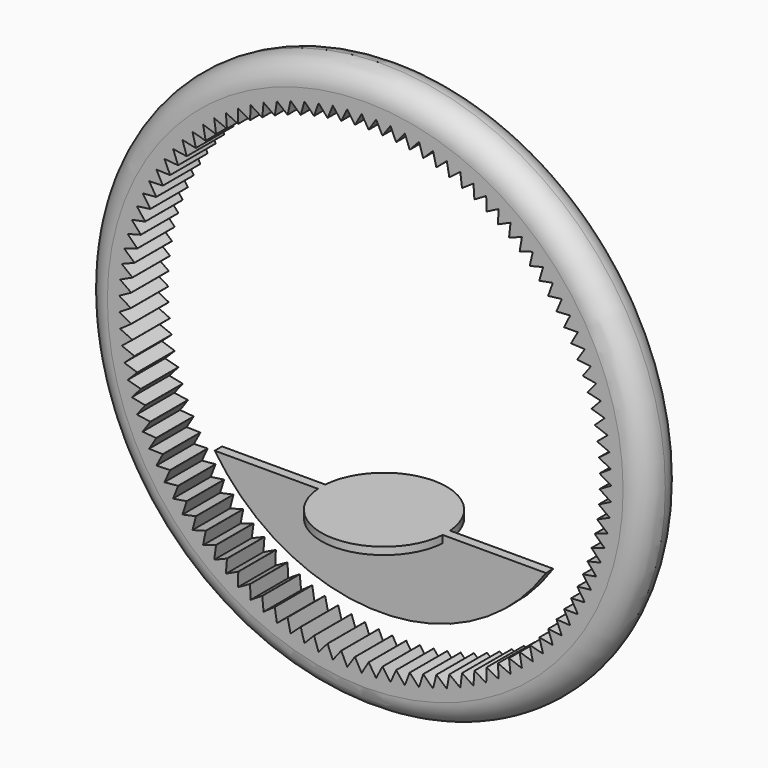
from build123d import *

# Parameters (mm, degrees)
F0_R          = 152.4
F1_DEPTH      = 12.7
F1_DEPTH_BACK = 12.7
F2_R          = 12.69999
F4_DEPTH      = 2.5
F6_DEPTH      = 4


# Not quite as in the source:
# - a fillet or chamfer is up to 0.001 mm smaller than in the source, because OpenCascade refuses the exact size


with BuildPart() as f1:
    # F0 (on Front) → F1 (new body, two sides)
    with BuildSketch(Plane.XZ) as f1_sk:
        Circle(F0_R)
        with BuildLine():
            ThreePointArc((126.9443490301, 3.7592884063), (126.9452637908, 3.7282705209), (126.9461709726, 3.6972524128))
            Line((126.9461709726, 3.6972524128), (133.35, 0))
            Line((133.35, 0), (126.9461709726, -3.6972524128))
            ThreePointArc((126.9461709726, -3.6972524128), (126.9452637908, -3.7282705209), (126.9443490301, -3.7592884063))
            Line((126.9443490301, -3.7592884063), (133.1201574625, -7.825993685))
            Line((133.1201574625, -7.825993685), (126.5103831653, -11.141048037))
            ThreePointArc((126.5103831653, -11.141048037), (126.5076571684, -11.1719594418), (126.5049236186, -11.2028701796))
            Line((126.5049236186, -11.2028701796), (132.4314221649, -15.6250095484))
            Line((132.4314221649, -15.6250095484), (125.6384878592, -18.5464381606))
            ThreePointArc((125.6384878592, -18.5464381606), (125.6339524441, -18.5771363041), (125.6294095284, -18.6078333386))
            Line((125.6294095284, -18.6078333386), (131.2861683203, -23.3701627671))
            Line((131.2861683203, -23.3701627671), (124.333490658, -25.8878948698))
            ThreePointArc((124.333490658, -25.8878948698), (124.3271614593, -25.9182739292), (124.3208248379, -25.9486514412))
            Line((124.3208248379, -25.9486514412), (129.6883438562, -31.0347541933))
            Line((129.6883438562, -31.0347541933), (122.5998901574, -33.1401106423))
            ThreePointArc((122.5998901574, -33.1401106423), (122.5917889932, -33.1700658947), (122.5836805098, -33.2000191667))
            Line((122.5836805098, -33.2000191667), (127.6434568043, -38.5923623926))
            Line((127.6434568043, -38.5923623926), (120.4436624375, -40.2780855882))
            ThreePointArc((120.4436624375, -40.2780855882), (120.433817234, -40.3075137715), (120.4239648403, -40.3369395484))
            Line((120.4239648403, -40.3369395484), (125.158556314, -46.0169347239))
            Line((125.158556314, -46.0169347239), (117.8722404618, -47.2772136289))
            ThreePointArc((117.8722404618, -47.2772136289), (117.8606851576, -47.3060132982), (117.8491228169, -47.3348101432))
            Line((117.8491228169, -47.3348101432), (122.2422083521, -53.2828771483))
            Line((122.2422083521, -53.2828771483), (114.8944884547, -54.1133673203))
            ThreePointArc((114.8944884547, -54.1133673203), (114.8812628833, -54.1414391971), (114.8680304533, -54.1695078415))
            Line((114.8680304533, -54.1695078415), (118.9044661741, -60.3651424569))
            Line((118.9044661741, -60.3651424569), (111.5206713441, -60.7629810242))
            ThreePointArc((111.5206713441, -60.7629810242), (111.5058210969, -60.790228339), (111.4909641924, -60.8174720244))
            Line((111.4909641924, -60.8174720244), (115.1568356688, -67.2393166142))
            Line((115.1568356688, -67.2393166142), (107.7624193767, -67.2031321449))
            ThreePointArc((107.7624193767, -67.2031321449), (107.7459956454, -67.2294609705), (107.7295654814, -67.2557857823))
            Line((107.7295654814, -67.2557857823), (111.0122356949, -73.8817029178))
            Line((111.0122356949, -73.8817029178), (103.6326880254, -73.4116201471))
            ThreePointArc((103.6326880254, -73.4116201471), (103.6147474261, -73.4369397226), (103.5968006407, -73.4622549137))
            Line((103.5968006407, -73.4622549137), (106.484953547, -80.2694036859))
            Line((106.484953547, -80.2694036859), (99.1457133298, -79.3670430866))
            ThreePointArc((99.1457133298, -79.3670430866), (99.1263177075, -79.3912661302), (99.106916167, -79.4154844339))
            Line((99.106916167, -79.4154844339), (101.5905957048, -86.3803991908))
            Line((101.5905957048, -86.3803991908), (94.3169628212, -85.0488713869))
            ThreePointArc((94.3169628212, -85.0488713869), (94.2961790365, -85.0719143966), (94.2753896221, -85.0949523274))
            Line((94.2753896221, -85.0949523274), (96.3460340334, -92.1936235649))
            Line((96.3460340334, -92.1936235649), (89.1630822029, -90.4375186086))
            ThreePointArc((89.1630822029, -90.4375186086), (89.1409819019, -90.4593021505), (89.1188762789, -90.4810802918))
            Line((89.1188762789, -90.4810802918), (90.7693476236, -97.6890374197))
            Line((90.7693476236, -97.6890374197), (83.7018379691, -95.5144089684))
            ThreePointArc((83.7018379691, -95.5144089684), (83.6784973361, -95.5348579502), (83.6551517073, -95.5553012283))
            Line((83.6551517073, -95.5553012283), (84.8797604686, -102.8476969251))
            Line((84.8797604686, -102.8476969251), (77.95205616, -100.2620413737))
            ThreePointArc((77.95205616, -100.2620413737), (77.927555655, -100.2810853034), (77.9030504975, -100.3001232461))
            Line((77.9030504975, -100.3001232461), (78.6975751954, -107.6518191131))
            Line((78.6975751954, -107.6518191131), (71.9335574647, -104.6640497519))
            ThreePointArc((71.9335574647, -104.6640497519), (71.907981546, -104.6816229812), (71.8824013342, -104.6991899607))
            Line((71.8824013342, -104.6991899607), (72.2441030774, -112.0848431793))
            Line((72.2441030774, -112.0848431793), (65.6670888949, -108.7052594683))
            ThreePointArc((65.6670888949, -108.7052594683), (65.640525728, -108.7213014186), (65.6139586422, -108.7373368779))
            Line((65.6139586422, -108.7373368779), (65.5415905699, -116.1314875715))
            Line((65.5415905699, -116.1314875715), (59.174252266, -112.3717396357))
            ThreePointArc((59.174252266, -112.3717396357), (59.1467934197, -112.3861950071), (59.1193310421, -112.4006436687))
            Line((59.1193310421, -112.4006436687), (58.6131426221, -119.777802668))
            Line((58.6131426221, -119.777802668), (52.477429731, -115.6508511375))
            ThreePointArc((52.477429731, -115.6508511375), (52.4491698615, -115.6636700993), (52.4209068606, -115.6764821557))
            Line((52.4209068606, -115.6764821557), (51.4826430292, -123.0112188653))
            Line((51.4826430292, -123.0112188653), (45.5997066243, -118.531290197))
            ThreePointArc((45.5997066243, -118.531290197), (45.5707431493, -118.5424285597), (45.5417769536, -118.5535598449))
            Line((45.5417769536, -118.5535598449), (44.1746721006, -125.820589908))
            Line((44.1746721006, -125.820589908), (38.5647918824, -121.0031273442))
            ThreePointArc((38.5647918824, -121.0031273442), (38.535224645, -121.0125467113), (38.5056551069, -121.0219588537))
            Line((38.5056551069, -121.0219588537), (36.714421926, -128.1962313122))
            Line((36.714421926, -128.1962313122), (31.3969363138, -123.0578416441))
            ThreePointArc((31.3969363138, -123.0578416441), (31.3668672383, -123.0655095453), (31.3367962902, -123.0731700992))
            Line((31.3367962902, -123.0731700992), (29.1276095332, -130.1299537496))
            Line((29.1276095332, -130.1299537496), (24.1208490014, -124.6883500711))
            ThreePointArc((24.1208490014, -124.6883500711), (24.0903817423, -124.6942400735), (24.0599130449, -124.7001226313))
            Line((24.0599130449, -124.7001226313), (21.4403882362, -131.6150912786))
            Line((21.4403882362, -131.6150912786), (16.7616121256, -125.8890319247))
            ThreePointArc((16.7616121256, -125.8890319247), (16.7308517098, -125.8931237243), (16.7000902951, -125.8972080077))
            Line((16.7000902951, -125.8972080077), (13.6792574793, -132.6465243224))
            Line((13.6792574793, -132.6465243224), (9.3445945005, -126.655748206))
            ThreePointArc((9.3445945005, -126.655748206), (9.3136469654, -126.6580276974), (9.2826988744, -126.660299627))
            Line((9.2826988744, -126.660299627), (5.8709714881, -133.2206973176))
            Line((5.8709714881, -133.2206973176), (1.8953641223, -126.985855885))
            ThreePointArc((1.8953641223, -126.985855885), (1.8643361506, -126.9863152104), (1.8333080676, -126.9867669544))
            Line((1.8333080676, -126.9867669544), (-1.9575529581, -133.3356309709))
            Line((-1.9575529581, -133.3356309709), (-5.5603999687, -126.8782170122))
            ThreePointArc((-5.5603999687, -126.8782170122), (-5.5914014172, -126.8768545882), (-5.6224025318, -126.8754845893))
            Line((-5.6224025318, -126.8754845893), (-9.7793293137, -132.9909290823))
            Line((-9.7793293137, -132.9909290823), (-12.9969962092, -126.333202641))
            ThreePointArc((-12.9969962092, -126.333202641), (-13.027864266, -126.3300231642), (-13.058731545, -126.3268361451))
            Line((-13.058731545, -126.3268361451), (-17.5673942953, -132.1877799105))
            Line((-17.5673942953, -132.1877799105), (-20.3887891111, -125.352691549))
            ThreePointArc((-20.3887891111, -125.352691549), (-20.4194173678, -125.3477059796), (-20.4500444053, -125.3427129267))
            Line((-20.4500444053, -125.3427129267), (-25.2949008294, -130.9289520772))
            Line((-25.2949008294, -130.9289520772), (-27.7102976333, -123.940063761))
            ThreePointArc((-27.7102976333, -123.940063761), (-27.7405805078, -123.9332892854), (-27.7708617261, -123.9265074106))
            Line((-27.7708617261, -123.9265074106), (-32.9352106003, -129.2187850226))
            Line((-32.9352106003, -129.2187850226), (-34.936283019, -122.1001888975))
            ThreePointArc((-34.936283019, -122.1001888975), (-34.96611612, -122.0916488687), (-34.9959471334, -122.0831015507))
            Line((-34.9959471334, -122.0831015507), (-40.4619858773, -127.0631740469))
            Line((-40.4619858773, -127.0631740469), (-42.0418357997, -119.8394093885))
            ThreePointArc((-42.0418357997, -119.8394093885), (-42.0711162863, -119.8291332457), (-42.1003942611, -119.8188499488))
            Line((-42.1003942611, -119.8188499488), (-47.8492803068, -124.4695499876))
            Line((-47.8492803068, -124.4695499876), (-49.0024616629, -117.1655186092))
            ThreePointArc((-49.0024616629, -117.1655186092), (-49.0310885993, -117.1535417765), (-49.0597126083, -117.1415579493))
            Line((-49.0597126083, -117.1415579493), (-55.0716283545, -121.4468536043))
            Line((-55.0716283545, -121.4468536043), (-55.7941658894, -114.0877340151))
            ThreePointArc((-55.7941658894, -114.0877340151), (-55.8220405925, -114.074097779), (-55.8499119628, -114.0604547323))
            Line((-55.8499119628, -114.0604547323), (-62.1041330907, -118.0055047574))
            Line((-62.1041330907, -118.0055047574), (-62.3935360677, -110.6166653673))
            ThreePointArc((-62.3935360677, -110.6166653673), (-62.4205624476, -110.6014167347), (-62.4475851008, -110.586161499))
            Line((-62.4475851008, -110.586161499), (-68.9225520144, -114.1573664895))
            Line((-68.9225520144, -114.1573664895), (-68.7778228015, -106.7642781584))
            ThreePointArc((-68.7778228015, -106.7642781584), (-68.8039076928, -106.7474696946), (-68.8299884762, -106.7306548577))
            Line((-68.8299884762, -106.7306548577), (-75.5033806233, -109.9157041303))
            Line((-75.5033806233, -109.9157041303), (-74.9250181321, -102.5438523652))
            ThreePointArc((-74.9250181321, -102.5438523652), (-74.9500716147, -102.5255420125), (-74.9751206225, -102.5072255387))
            Line((-74.9751206225, -102.5072255387), (-81.8239334378, -105.2951395686))
            Line((-81.8239334378, -105.2951395686), (-80.8139314036, -97.9699366699))
            ThreePointArc((-80.8139314036, -97.9699366699), (-80.8378671129, -97.9501875477), (-80.861797996, -97.9304325777))
            Line((-80.861797996, -97.9304325777), (-87.8624222029, -100.3116008477))
            Line((-87.8624222029, -100.3116008477), (-86.424262312, -93.0582983072))
            ThreePointArc((-86.424262312, -93.0582983072), (-86.4469977367, -93.037178495), (-86.4697280003, -93.0160531282))
            Line((-86.4697280003, -93.0160531282), (-93.598030997, -94.9822672581))
            Line((-93.598030997, -94.9822672581), (-91.7366708844, -87.8258687121))
            ThreePointArc((-91.7366708844, -87.8258687121), (-91.7581276509, -87.8034510142), (-91.7795789391, -87.7810280742))
            Line((-91.7795789391, -87.7810280742), (-99.0109879884, -89.3255101165))
            Line((-99.0109879884, -89.3255101165), (-96.732844148, -82.2906851535))
            ThreePointArc((-96.732844148, -82.2906851535), (-96.7529482902, -82.2670468483), (-96.773046656, -82.2434036316))
            Line((-96.773046656, -82.2434036316), (-104.0826335929, -83.3608294367))
            Line((-104.0826335929, -83.3608294367), (-101.3955592585, -76.4718285557))
            ThreePointArc((-101.3955592585, -76.4718285557), (-101.4142414734, -76.4470511294), (-101.4329176335, -76.422269139))
            Line((-101.4329176335, -76.422269139), (-108.7954847974, -77.1087867087))
            Line((-108.7954847974, -77.1087867087), (-105.708742871, -70.3893577228))
            ThreePointArc((-105.708742871, -70.3893577228), (-105.725938757, -70.3635265883), (-105.7431283309, -70.3376912529))
            Line((-105.7431283309, -70.3376912529), (-113.1332954277, -70.590934019))
            Line((-113.1332954277, -70.590934019), (-109.657526548, -64.0642401919))
            ThreePointArc((-109.657526548, -64.0642401919), (-109.6731768274, -64.0374443945), (-109.688820559, -64.0106447739))
            Line((-109.688820559, -64.0106447739), (-117.0811121517, -63.829739756))
            Line((-117.0811121517, -63.829739756), (-113.2282980142, -57.5182799535))
            ThreePointArc((-113.2282980142, -57.5182799535), (-113.2423487373, -57.4906118638), (-113.2563926994, -57.4629403417))
            Line((-113.2563926994, -57.4629403417), (-120.6253260275, -56.8485111569))
            Line((-120.6253260275, -56.8485111569), (-116.4087480806, -50.7740422884))
            ThreePointArc((-116.4087480806, -50.7740422884), (-116.4211508115, -50.7455972841), (-116.4335465918, -50.7171492501))
            Line((-116.4335465918, -50.7171492501), (-123.7537194155, -49.6713139631))
            Line((-123.7537194155, -49.6713139631), (-119.187913077, -43.8547759812))
            ThreePointArc((-119.187913077, -43.8547759812), (-119.198625061, -43.825652118), (-119.2093299285, -43.7965256384))
            Line((-119.2093299285, -43.7965256384), (-126.4555080957, -42.3228894601))
            Line((-126.4555080957, -42.3228894601), (-121.5562126458, -36.7843331761))
            ThreePointArc((-121.5562126458, -36.7843331761), (-121.5651969565, -36.7546308501), (-121.5741740094, -36.7249263298))
            Line((-121.5741740094, -36.7249263298), (-128.7213784428, -34.8285691894))
            Line((-128.7213784428, -34.8285691894), (-123.5054827679, -29.5870871543))
            ThreePointArc((-123.5054827679, -29.5870871543), (-123.5127084345, -29.5569087556), (-123.519926727, -29.5267285922))
            Line((-123.519926727, -29.5267285922), (-130.5435195323, -27.2141876256))
            Line((-130.5435195323, -27.2141876256), (-125.0290039053, -22.2878483137))
            ThreePointArc((-125.0290039053, -22.2878483137), (-125.0344460194, -22.2572978734), (-125.0398806686, -22.2267461044))
            Line((-125.0398806686, -22.2267461044), (-131.9156500664, -19.5059931194))
            Line((-131.9156500664, -19.5059931194), (-126.121524165, -14.9117786428))
            ThreePointArc((-126.121524165, -14.9117786428), (-126.1251639665, -14.8809614747), (-126.1287962381, -14.8501434182))
            Line((-126.1287962381, -14.8501434182), (-132.8330400268, -11.7305574139))
            Line((-132.8330400268, -11.7305574139), (-126.7792774034, -7.4843049818))
            ThreePointArc((-126.7792774034, -7.4843049818), (-126.7811023452, -7.453327319), (-126.7829197179, -7.4223492112))
            Line((-126.7829197179, -7.4223492112), (-133.2925269804, -3.9146840469))
            Line((-133.2925269804, -3.9146840469), (-126.9999962089, -0.0310313711))
            ThreePointArc((-126.9999962089, -0.0310313711), (-127, 0), (-126.9999962089, 0.0310313711))
            Line((-126.9999962089, 0.0310313711), (-133.2925269804, 3.9146840469))
            Line((-133.2925269804, 3.9146840469), (-126.7829197179, 7.4223492112))
            ThreePointArc((-126.7829197179, 7.4223492112), (-126.7811023452, 7.453327319), (-126.7792774034, 7.4843049818))
            Line((-126.7792774034, 7.4843049818), (-132.8330400268, 11.7305574139))
            Line((-132.8330400268, 11.7305574139), (-126.1287962381, 14.8501434182))
            ThreePointArc((-126.1287962381, 14.8501434182), (-126.1251639665, 14.8809614747), (-126.121524165, 14.9117786428))
            Line((-126.121524165, 14.9117786428), (-131.9156500664, 19.5059931194))
            Line((-131.9156500664, 19.5059931194), (-125.0398806686, 22.2267461044))
            ThreePointArc((-125.0398806686, 22.2267461044), (-125.0344460194, 22.2572978734), (-125.0290039053, 22.2878483137))
            Line((-125.0290039053, 22.2878483137), (-130.5435195323, 27.2141876256))
            Line((-130.5435195323, 27.2141876256), (-123.519926727, 29.5267285922))
            ThreePointArc((-123.519926727, 29.5267285922), (-123.5127084345, 29.5569087556), (-123.5054827679, 29.5870871543))
            Line((-123.5054827679, 29.5870871543), (-128.7213784428, 34.8285691894))
            Line((-128.7213784428, 34.8285691894), (-121.5741740094, 36.7249263298))
            ThreePointArc((-121.5741740094, 36.7249263298), (-121.5651969565, 36.7546308501), (-121.5562126458, 36.7843331761))
            Line((-121.5562126458, 36.7843331761), (-126.4555080957, 42.3228894601))
            Line((-126.4555080957, 42.3228894601), (-119.2093299285, 43.7965256384))
            ThreePointArc((-119.2093299285, 43.7965256384), (-119.198625061, 43.825652118), (-119.187913077, 43.8547759812))
            Line((-119.187913077, 43.8547759812), (-123.7537194155, 49.6713139631))
            Line((-123.7537194155, 49.6713139631), (-116.4335465918, 50.7171492501))
            ThreePointArc((-116.4335465918, 50.7171492501), (-116.4211508115, 50.7455972841), (-116.4087480806, 50.7740422884))
            Line((-116.4087480806, 50.7740422884), (-120.6253260275, 56.8485111569))
            Line((-120.6253260275, 56.8485111569), (-113.2563926994, 57.4629403417))
            ThreePointArc((-113.2563926994, 57.4629403417), (-113.2423487373, 57.4906118638), (-113.2282980142, 57.5182799535))
            Line((-113.2282980142, 57.5182799535), (-117.0811121517, 63.829739756))
            Line((-117.0811121517, 63.829739756), (-109.688820559, 64.0106447739))
            ThreePointArc((-109.688820559, 64.0106447739), (-109.6731768274, 64.0374443945), (-109.657526548, 64.0642401919))
            Line((-109.657526548, 64.0642401919), (-113.1332954277, 70.590934019))
            Line((-113.1332954277, 70.590934019), (-105.7431283309, 70.3376912529))
            ThreePointArc((-105.7431283309, 70.3376912529), (-105.725938757, 70.3635265883), (-105.708742871, 70.3893577228))
            Line((-105.708742871, 70.3893577228), (-108.7954847974, 77.1087867087))
            Line((-108.7954847974, 77.1087867087), (-101.4329176335, 76.422269139))
            ThreePointArc((-101.4329176335, 76.422269139), (-101.4142414734, 76.4470511294), (-101.3955592585, 76.4718285557))
            Line((-101.3955592585, 76.4718285557), (-104.0826335929, 83.3608294367))
            Line((-104.0826335929, 83.3608294367), (-96.773046656, 82.2434036316))
            ThreePointArc((-96.773046656, 82.2434036316), (-96.7529482902, 82.2670468483), (-96.732844148, 82.2906851535))
            Line((-96.732844148, 82.2906851535), (-99.0109879884, 89.3255101165))
            Line((-99.0109879884, 89.3255101165), (-91.7795789391, 87.7810280742))
            ThreePointArc((-91.7795789391, 87.7810280742), (-91.7581276509, 87.8034510142), (-91.7366708844, 87.8258687121))
            Line((-91.7366708844, 87.8258687121), (-93.598030997, 94.9822672581))
            Line((-93.598030997, 94.9822672581), (-86.4697280003, 93.0160531282))
            ThreePointArc((-86.4697280003, 93.0160531282), (-86.4469977367, 93.037178495), (-86.424262312, 93.0582983072))
            Line((-86.424262312, 93.0582983072), (-87.8624222029, 100.3116008477))
            Line((-87.8624222029, 100.3116008477), (-80.861797996, 97.9304325777))
            ThreePointArc((-80.861797996, 97.9304325777), (-80.8378671129, 97.9501875477), (-80.8139314036, 97.9699366699))
            Line((-80.8139314036, 97.9699366699), (-81.8239334378, 105.2951395686))
            Line((-81.8239334378, 105.2951395686), (-74.9751206225, 102.5072255387))
            ThreePointArc((-74.9751206225, 102.5072255387), (-74.9500716147, 102.5255420125), (-74.9250181321, 102.5438523652))
            Line((-74.9250181321, 102.5438523652), (-75.5033806233, 109.9157041303))
            Line((-75.5033806233, 109.9157041303), (-68.8299884762, 106.7306548577))
            ThreePointArc((-68.8299884762, 106.7306548577), (-68.8039076928, 106.7474696946), (-68.7778228015, 106.7642781584))
            Line((-68.7778228015, 106.7642781584), (-68.9225520144, 114.1573664895))
            Line((-68.9225520144, 114.1573664895), (-62.4475851008, 110.586161499))
            ThreePointArc((-62.4475851008, 110.586161499), (-62.4205624476, 110.6014167347), (-62.3935360677, 110.6166653673))
            Line((-62.3935360677, 110.6166653673), (-62.1041330907, 118.0055047574))
            Line((-62.1041330907, 118.0055047574), (-55.8499119628, 114.0604547323))
            ThreePointArc((-55.8499119628, 114.0604547323), (-55.8220405925, 114.074097779), (-55.7941658894, 114.0877340151))
            Line((-55.7941658894, 114.0877340151), (-55.0716283545, 121.4468536043))
            Line((-55.0716283545, 121.4468536043), (-49.0597126083, 117.1415579493))
            ThreePointArc((-49.0597126083, 117.1415579493), (-49.0310885993, 117.1535417765), (-49.0024616629, 117.1655186092))
            Line((-49.0024616629, 117.1655186092), (-47.8492803068, 124.4695499876))
            Line((-47.8492803068, 124.4695499876), (-42.1003942611, 119.8188499488))
            ThreePointArc((-42.1003942611, 119.8188499488), (-42.0711162863, 119.8291332457), (-42.0418357997, 119.8394093885))
            Line((-42.0418357997, 119.8394093885), (-40.4619858773, 127.0631740469))
            Line((-40.4619858773, 127.0631740469), (-34.9959471334, 122.0831015507))
            ThreePointArc((-34.9959471334, 122.0831015507), (-34.96611612, 122.0916488687), (-34.936283019, 122.1001888975))
            Line((-34.936283019, 122.1001888975), (-32.9352106003, 129.2187850226))
            Line((-32.9352106003, 129.2187850226), (-27.7708617261, 123.9265074106))
            ThreePointArc((-27.7708617261, 123.9265074106), (-27.7405805078, 123.9332892854), (-27.7102976333, 123.940063761))
            Line((-27.7102976333, 123.940063761), (-25.2949008294, 130.9289520772))
            Line((-25.2949008294, 130.9289520772), (-20.4500444053, 125.3427129267))
            ThreePointArc((-20.4500444053, 125.3427129267), (-20.4194173678, 125.3477059796), (-20.3887891111, 125.352691549))
            Line((-20.3887891111, 125.352691549), (-17.5673942953, 132.1877799105))
            Line((-17.5673942953, 132.1877799105), (-13.058731545, 126.3268361451))
            ThreePointArc((-13.058731545, 126.3268361451), (-13.027864266, 126.3300231642), (-12.9969962092, 126.333202641))
            Line((-12.9969962092, 126.333202641), (-9.7793293137, 132.9909290823))
            Line((-9.7793293137, 132.9909290823), (-5.6224025318, 126.8754845893))
            ThreePointArc((-5.6224025318, 126.8754845893), (-5.5914014172, 126.8768545882), (-5.5603999687, 126.8782170122))
            Line((-5.5603999687, 126.8782170122), (-1.9575529581, 133.3356309709))
            Line((-1.9575529581, 133.3356309709), (1.8333080676, 126.9867669544))
            ThreePointArc((1.8333080676, 126.9867669544), (1.8643361506, 126.9863152104), (1.8953641223, 126.985855885))
            Line((1.8953641223, 126.985855885), (5.8709714881, 133.2206973176))
            Line((5.8709714881, 133.2206973176), (9.2826988744, 126.660299627))
            ThreePointArc((9.2826988744, 126.660299627), (9.3136469654, 126.6580276974), (9.3445945005, 126.655748206))
            Line((9.3445945005, 126.655748206), (13.6792574793, 132.6465243224))
            Line((13.6792574793, 132.6465243224), (16.7000902951, 125.8972080077))
            ThreePointArc((16.7000902951, 125.8972080077), (16.7308517098, 125.8931237243), (16.7616121256, 125.8890319247))
            Line((16.7616121256, 125.8890319247), (21.4403882362, 131.6150912786))
            Line((21.4403882362, 131.6150912786), (24.0599130449, 124.7001226313))
            ThreePointArc((24.0599130449, 124.7001226313), (24.0903817423, 124.6942400735), (24.1208490014, 124.6883500711))
            Line((24.1208490014, 124.6883500711), (29.1276095332, 130.1299537496))
            Line((29.1276095332, 130.1299537496), (31.3367962902, 123.0731700992))
            ThreePointArc((31.3367962902, 123.0731700992), (31.3668672383, 123.0655095453), (31.3969363138, 123.0578416441))
            Line((31.3969363138, 123.0578416441), (36.714421926, 128.1962313122))
            Line((36.714421926, 128.1962313122), (38.5056551069, 121.0219588537))
            ThreePointArc((38.5056551069, 121.0219588537), (38.535224645, 121.0125467113), (38.5647918824, 121.0031273442))
            Line((38.5647918824, 121.0031273442), (44.1746721006, 125.820589908))
            Line((44.1746721006, 125.820589908), (45.5417769536, 118.5535598449))
            ThreePointArc((45.5417769536, 118.5535598449), (45.5707431493, 118.5424285597), (45.5997066243, 118.531290197))
            Line((45.5997066243, 118.531290197), (51.4826430292, 123.0112188653))
            Line((51.4826430292, 123.0112188653), (52.4209068606, 115.6764821557))
            ThreePointArc((52.4209068606, 115.6764821557), (52.4491698615, 115.6636700993), (52.477429731, 115.6508511375))
            Line((52.477429731, 115.6508511375), (58.6131426221, 119.777802668))
            Line((58.6131426221, 119.777802668), (59.1193310421, 112.4006436687))
            ThreePointArc((59.1193310421, 112.4006436687), (59.1467934197, 112.3861950071), (59.174252266, 112.3717396357))
            Line((59.174252266, 112.3717396357), (65.5415905699, 116.1314875715))
            Line((65.5415905699, 116.1314875715), (65.6139586422, 108.7373368779))
            ThreePointArc((65.6139586422, 108.7373368779), (65.640525728, 108.7213014186), (65.6670888949, 108.7052594683))
            Line((65.6670888949, 108.7052594683), (72.2441030774, 112.0848431793))
            Line((72.2441030774, 112.0848431793), (71.8824013342, 104.6991899607))
            ThreePointArc((71.8824013342, 104.6991899607), (71.907981546, 104.6816229812), (71.9335574647, 104.6640497519))
            Line((71.9335574647, 104.6640497519), (78.6975751954, 107.6518191131))
            Line((78.6975751954, 107.6518191131), (77.9030504975, 100.3001232461))
            ThreePointArc((77.9030504975, 100.3001232461), (77.927555655, 100.2810853034), (77.95205616, 100.2620413737))
            Line((77.95205616, 100.2620413737), (84.8797604686, 102.8476969251))
            Line((84.8797604686, 102.8476969251), (83.6551517073, 95.5553012283))
            ThreePointArc((83.6551517073, 95.5553012283), (83.6784973361, 95.5348579502), (83.7018379691, 95.5144089684))
            Line((83.7018379691, 95.5144089684), (90.7693476236, 97.6890374197))
            Line((90.7693476236, 97.6890374197), (89.1188762789, 90.4810802918))
            ThreePointArc((89.1188762789, 90.4810802918), (89.1409819019, 90.4593021505), (89.1630822029, 90.4375186086))
            Line((89.1630822029, 90.4375186086), (96.3460340334, 92.1936235649))
            Line((96.3460340334, 92.1936235649), (94.2753896221, 85.0949523274))
            ThreePointArc((94.2753896221, 85.0949523274), (94.2961790365, 85.0719143966), (94.3169628212, 85.0488713869))
            Line((94.3169628212, 85.0488713869), (101.5905957048, 86.3803991908))
            Line((101.5905957048, 86.3803991908), (99.106916167, 79.4154844339))
            ThreePointArc((99.106916167, 79.4154844339), (99.1263177075, 79.3912661302), (99.1457133298, 79.3670430866))
            Line((99.1457133298, 79.3670430866), (106.484953547, 80.2694036859))
            Line((106.484953547, 80.2694036859), (103.5968006407, 73.4622549137))
            ThreePointArc((103.5968006407, 73.4622549137), (103.6147474261, 73.4369397226), (103.6326880254, 73.4116201471))
            Line((103.6326880254, 73.4116201471), (111.0122356949, 73.8817029178))
            Line((111.0122356949, 73.8817029178), (107.7295654814, 67.2557857823))
            ThreePointArc((107.7295654814, 67.2557857823), (107.7459956454, 67.2294609705), (107.7624193767, 67.2031321449))
            Line((107.7624193767, 67.2031321449), (115.1568356688, 67.2393166142))
            Line((115.1568356688, 67.2393166142), (111.4909641924, 60.8174720244))
            ThreePointArc((111.4909641924, 60.8174720244), (111.5058210969, 60.790228339), (111.5206713441, 60.7629810242))
            Line((111.5206713441, 60.7629810242), (118.9044661741, 60.3651424569))
            Line((118.9044661741, 60.3651424569), (114.8680304533, 54.1695078415))
            ThreePointArc((114.8680304533, 54.1695078415), (114.8812628833, 54.1414391971), (114.8944884547, 54.1133673203))
            Line((114.8944884547, 54.1133673203), (122.2422083521, 53.2828771483))
            Line((122.2422083521, 53.2828771483), (117.8491228169, 47.3348101432))
            ThreePointArc((117.8491228169, 47.3348101432), (117.8606851576, 47.3060132982), (117.8722404618, 47.2772136289))
            Line((117.8722404618, 47.2772136289), (125.158556314, 46.0169347239))
            Line((125.158556314, 46.0169347239), (120.4239648403, 40.3369395484))
            ThreePointArc((120.4239648403, 40.3369395484), (120.433817234, 40.3075137715), (120.4436624375, 40.2780855882))
            Line((120.4436624375, 40.2780855882), (127.6434568043, 38.5923623926))
            Line((127.6434568043, 38.5923623926), (122.5836805098, 33.2000191667))
            ThreePointArc((122.5836805098, 33.2000191667), (122.5917889932, 33.1700658947), (122.5998901574, 33.1401106423))
            Line((122.5998901574, 33.1401106423), (129.6883438562, 31.0347541933))
            Line((129.6883438562, 31.0347541933), (124.3208248379, 25.9486514412))
            ThreePointArc((124.3208248379, 25.9486514412), (124.3271614593, 25.9182739292), (124.333490658, 25.8878948698))
            Line((124.333490658, 25.8878948698), (131.2861683203, 23.3701627671))
            Line((131.2861683203, 23.3701627671), (125.6294095284, 18.6078333386))
            ThreePointArc((125.6294095284, 18.6078333386), (125.6339524441, 18.5771363041), (125.6384878592, 18.5464381606))
            Line((125.6384878592, 18.5464381606), (132.4314221649, 15.6250095484))
            Line((132.4314221649, 15.6250095484), (126.5049236186, 11.2028701796))
            ThreePointArc((126.5049236186, 11.2028701796), (126.5076571684, 11.1719594418), (126.5103831653, 11.141048037))
            Line((126.5103831653, 11.141048037), (133.1201574625, 7.825993685))
            Line((133.1201574625, 7.825993685), (126.9443490301, 3.7592884063))
        make_face(mode=Mode.SUBTRACT)
    extrude(amount=F1_DEPTH)
    extrude(f1_sk.sketch, amount=-F1_DEPTH_BACK)

    # F2 (radius 12.7 in the source; OpenCascade refuses exactly that, so slightly less here)
    f2_edges = [f1.edges().sort_by_distance(p)[0] for p in [
        (152.4, -6.35, 0),
        (-152.4, 0, 0),
        (-152.4, -12.7, 0),
        (-152.4, 12.7, 0),
    ]]
    fillet(f2_edges, radius=F2_R)


with BuildPart() as f4:
    # F3 (on Front) → F4 (new body, symmetric)
    with BuildSketch(Plane.XZ):
        with BuildLine():
            Line((89.7117396298, -60), (-89.7117396298, -60))
            ThreePointArc((-89.7117396298, -60), (0, -107.926809586), (89.7117396298, -60))
        make_face()
    extrude(amount=F4_DEPTH, both=True)

    # F5 (on face) → F6 (join)
    with BuildSketch(Plane.XY.offset(-60)):
        with BuildLine():
            Line((-33.8211942774, 2.5), (33.8211942774, 2.5))
            ThreePointArc((33.8211942774, 2.5), (0, 33.9134660917), (-33.8211942774, 2.5))
        make_face()
        with BuildLine():
            ThreePointArc((33.8211942774, -2.5), (33.8903902873, -1.250851119), (33.9134660917, 0))
            ThreePointArc((33.9134660917, 0), (33.8903902873, 1.250851119), (33.8211942774, 2.5))
            Line((33.8211942774, 2.5), (-33.8211942774, 2.5))
            ThreePointArc((-33.8211942774, 2.5), (-33.9134660917, 0), (-33.8211942774, -2.5))
            Line((-33.8211942774, -2.5), (33.8211942774, -2.5))
        make_face()
        with BuildLine():
            ThreePointArc((-33.8211942774, -2.5), (0, -33.9134660917), (33.8211942774, -2.5))
            Line((33.8211942774, -2.5), (-33.8211942774, -2.5))
        make_face()
    extrude(amount=-F6_DEPTH)


solid = Compound([f1.part, f4.part])
